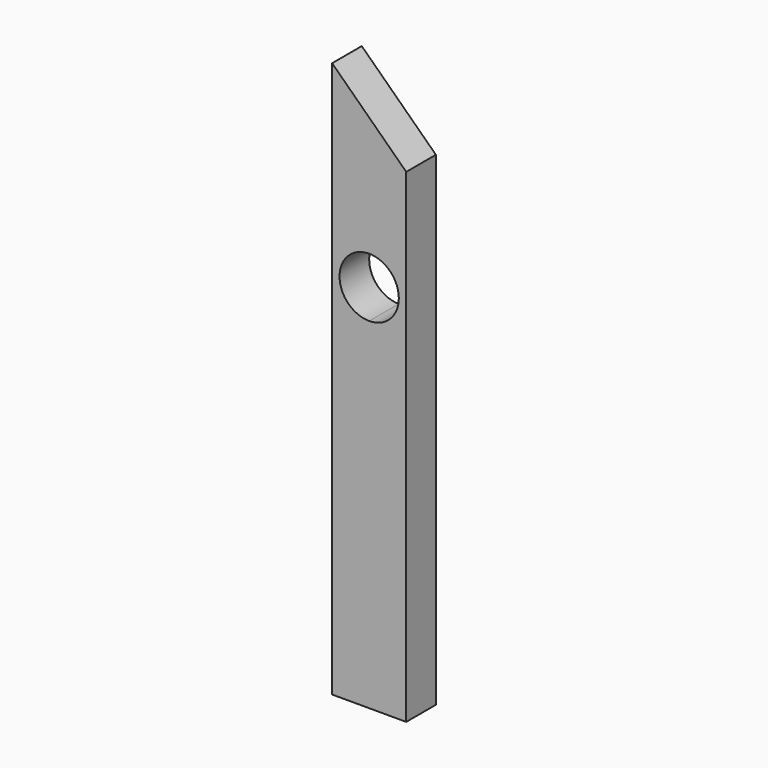
from build123d import *

# Parameters (mm, degrees)
F0_W     = 5.08
F0_H     = 38.1
F1_DEPTH = 2.54
F2_SIZE2 = 4.905689
F2_SIZE  = 5.07999
F4_DEPTH = 25.4


# Not quite as in the source:
# - a fillet or chamfer is up to 0.001 mm smaller than in the source, because OpenCascade refuses the exact size


with BuildPart() as f1:
    # F0 (on Front) → F1 (new body)
    with BuildSketch(Plane.XZ):
        Rectangle(F0_W, F0_H)
    extrude(amount=F1_DEPTH)

    # F2 (size 5.08 and 4.905698976 in the source; OpenCascade refuses exactly that, so slightly less here)
    f2_edges = [f1.edges().sort_by_distance(p)[0] for p in [
        (2.54, -1.27, 19.05),
    ]]
    f2_side = f1.faces().sort_by_distance((0, -1.27, 19.05))[0]
    chamfer(f2_edges, length=F2_SIZE, length2=F2_SIZE2, reference=f2_side)

    # F3 (on face) → F4 (cut)
    with BuildSketch(Plane.XZ.offset(2.54)):
        with BuildLine():
            ThreePointArc((0, 4.318), (1.4368409794, 4.9131590206), (2.032, 6.35))
            ThreePointArc((2.032, 6.35), (-1.4368409794, 7.7868409794), (0, 4.318))
        make_face()
    extrude(amount=-F4_DEPTH, mode=Mode.SUBTRACT)


solid = f1.part
